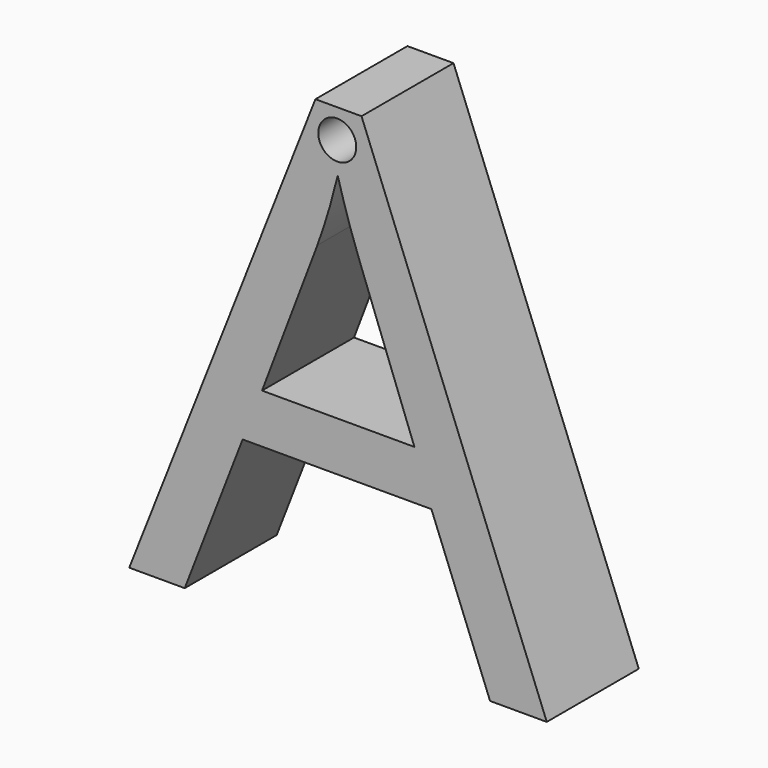
from build123d import *

# Parameters (mm, degrees)
F0_TEXT_SIZE = 145.7377026478
F1_DEPTH     = 25.4
F2_R         = 4.1949637234
F3_DEPTH     = 25.4


# Not quite as in the source:
# - Text() gives the source's letters only with a copy of the font that has no kerning and outlines rounded to 1/6400 em; it was checked with that copy


with BuildPart() as f1:
    # F0 (on Front) → F1 (new body)
    with BuildSketch(Plane.XZ):
        with Locations((-59.9318295717, -48.3288653195)):
            Text('A', F0_TEXT_SIZE, font='Open Sans', text_align=(TextAlign.LEFT, TextAlign.BOTTOM))
    extrude(amount=F1_DEPTH)

    # F2 (on Front) → F3 (cut)
    with BuildSketch(Plane.XZ):
        with Locations((-13.9853786677, 49.7710593045)):
            Circle(F2_R)
    extrude(amount=F3_DEPTH, mode=Mode.SUBTRACT)


solid = f1.part
